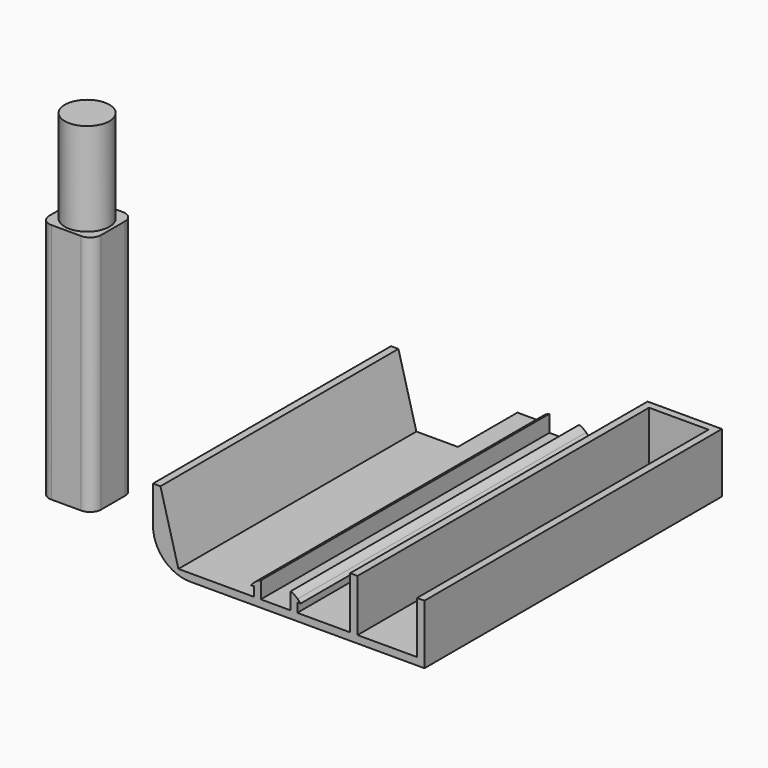
from build123d import *

# Parameters (mm, degrees)
F0_W           = 55
F0_H           = 100
F1_DEPTH       = 2
F2_W           = 16
F2_H           = 2
F3_DEPTH       = 14
F4_W           = 1.8
F4_H           = 100
F5_DEPTH       = 2.5
F7_W           = 1.8
F7_H           = 100
F7_W_2         = 0.9
F6_W           = 1.8
F6_H           = 100
F6_W_2         = 0.9
F8_DEPTH       = 2
F9_SIZE        = 1.99999
F10_T1_DEPTH   = 108.3703792641
F11_W          = 5
F11_H          = 3
F11_W_2        = 8
F12_DEPTH      = 2.001
F12_DEPTH_BACK = 10
F13_W          = 14
F13_H          = 14
F15_DEPTH      = 65
F16_R          = 6
F17_DEPTH      = 25
F18_R          = 3
F19_R          = 1.5
F20_DEPTH      = 30
F21_W          = 18
F21_H          = 80
F22_DEPTH      = 20
F23_T4_DEPTH   = 390.1150986591
F24_R          = 10


# Not quite as in the source:
# - a fillet or chamfer that OpenCascade refuses, or shapes differently, is made with other operations: its cross-section is extruded or revolved along the edge and cut away or added
# - a fillet or chamfer is up to 0.001 mm smaller than in the source, because OpenCascade refuses the exact size


with BuildPart() as f1:
    # F0 (on Top) → F1 (new body)
    with BuildSketch(Plane.XY):
        with Locations((27.5, 50)):
            Rectangle(F0_W, F0_H)
    extrude(amount=F1_DEPTH)

    # F2 (on face) → F3 (join)
    with BuildSketch(Plane.XY.offset(2)):
        Polygon((37, 98), (37, 100), (35, 100), (35, 0), (37, 0), align=None)
        Polygon((55, 0), (55, 100), (53, 100), (53, 98), (53, 0), align=None)
        with Locations((45, 99)):
            Rectangle(F2_W, F2_H)
    extrude(amount=F3_DEPTH)

    # F4 (on face) → F5 (join)
    with BuildSketch(Plane.XY.offset(2)):
        with Locations((10.1, 50)):
            Rectangle(F4_W, F4_H)
        with Locations((19.9, 50)):
            Rectangle(F4_W, F4_H)
    extrude(amount=F5_DEPTH)

    # F7 (on face) + F6 (on face) → F8 (join)
    with BuildSketch(Plane.XY.offset(4.5)):
        with Locations((19.9, 50)):
            Rectangle(F7_W, F7_H)
        with Locations((21.25, 50)):
            Rectangle(F7_W_2, F7_H)
    with BuildSketch(Plane.XY.offset(4.5)):
        with Locations((10.1, 50)):
            Rectangle(F6_W, F6_H)
        with Locations((8.75, 50)):
            Rectangle(F6_W_2, F6_H)
    extrude(amount=F8_DEPTH)

    # F9 (size 2 in the source; OpenCascade refuses exactly that, so slightly less here)
    f9_edges = [f1.edges().sort_by_distance(p)[0] for p in [
        (8.3, 50, 6.5),
        (21.7, 50, 6.5),
    ]]
    chamfer(f9_edges, length=F9_SIZE)

    # F10: fillet of radius 5 on 2 edges, made by hand

    # F10_s2 → F10_t1 (cut)
    with BuildSketch(Plane.XZ.offset(-104.1851896321)):
        with BuildLine():
            ThreePointArc((9.1162396122, 5.3162496122), (9.9914434967, 6.0142301065), (11, 6.5))
            Line((11, 6.5), (10.29999, 6.5))
            Line((10.29999, 6.5), (9.1162396122, 5.3162496122))
        make_face()
        with BuildLine():
            ThreePointArc((20.8837603878, 5.3162496122), (20.0085565033, 6.0142301065), (19, 6.5))
            Line((19, 6.5), (19.70001, 6.5))
            Line((19.70001, 6.5), (20.8837603878, 5.3162496122))
        make_face()
    extrude(amount=F10_T1_DEPTH, mode=Mode.SUBTRACT)

    # F11 (on face) → F12 (cut, two sides)
    with BuildSketch(Plane.XY.offset(2)) as f12_sk:
        with Locations((8.5, 98.5)):
            Rectangle(F11_W, F11_H)
        with Locations((15, 98.5)):
            Rectangle(F11_W_2, F11_H)
        with Locations((21.5, 98.5)):
            Rectangle(F11_W, F11_H)
    extrude(amount=-F12_DEPTH, mode=Mode.SUBTRACT)
    extrude(f12_sk.sketch, amount=F12_DEPTH_BACK, mode=Mode.SUBTRACT)

    # F21 (on Top) → F22 (join)
    with BuildSketch(Plane.XY):
        with Locations((-9, 40)):
            Rectangle(F21_W, F21_H)
    extrude(amount=F22_DEPTH)

    # F23: chamfer of 16 x 59.7128129211 on 1 edges, made by hand


with BuildPart() as f15:
    # F13 (on Top) → F15 (new body)
    with BuildSketch(Plane.XY):
        with Locations((-50.0888161063, 17.9589258209)):
            Rectangle(F13_W, F13_H)
    extrude(amount=F15_DEPTH)

    # F16 (on face) → F17 (join)
    with BuildSketch(Plane.XY.offset(65)):
        with Locations((-50.0888161063, 17.9589258209)):
            Circle(F16_R)
    extrude(amount=F17_DEPTH)

    # F18
    f18_edges = [f15.edges().sort_by_distance(p)[0] for p in [
        (-57.088816, 10.958926, 32.5),
        (-43.088816, 10.958926, 32.5),
        (-43.088816, 24.958926, 32.5),
        (-57.088816, 24.958926, 32.5),
    ]]
    fillet(f18_edges, radius=F18_R)

    # F19 (on face) → F20 (cut)
    with BuildSketch(Plane.XY):
        with Locations((-50.0888161063, 17.9589258209)):
            Circle(F19_R)
    extrude(amount=F20_DEPTH, mode=Mode.SUBTRACT)


with BuildPart() as f23_tool2:
    # F23_s3 → F23_t4 (new body)
    with BuildSketch(Plane.XZ.offset(155.0575493296)):
        Polygon((0, -39.7128129211), (-16, 20), (0, 20), align=None)
    extrude(amount=-F23_T4_DEPTH)

    split(bisect_by=Plane.XY.offset(2), keep=Keep.TOP)


with BuildPart() as f1_1:
    add(f1.part)

    # F23_t1: cut F23_tool2
    add(f23_tool2.part, mode=Mode.SUBTRACT)

    # F24
    f24_edges = [f1_1.edges().sort_by_distance(p)[0] for p in [
        (-18, 40, 0),
    ]]
    fillet(f24_edges, radius=F24_R)


solid = Compound([f15.part, f1_1.part])
